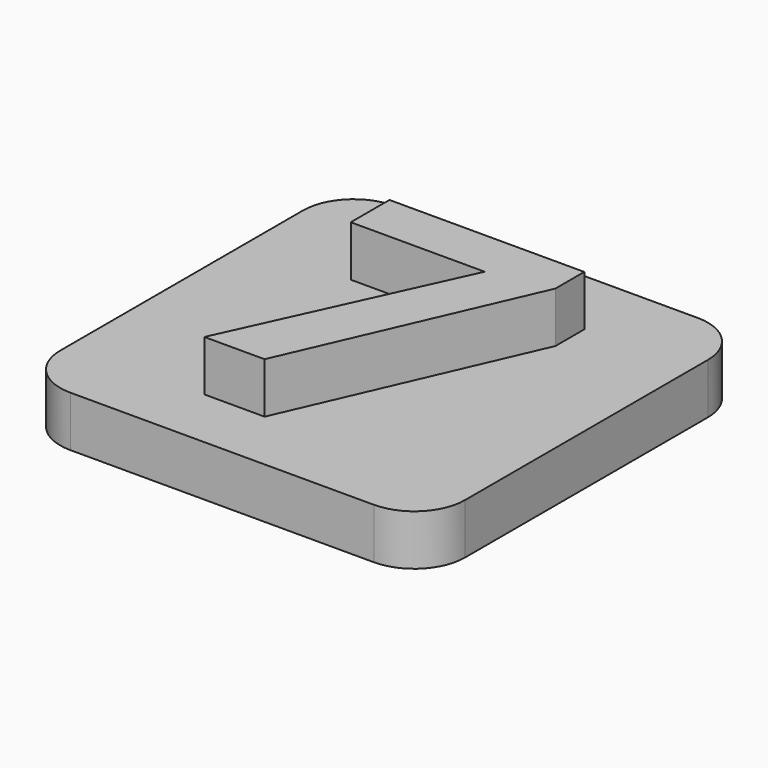
from build123d import *

# Parameters (mm, degrees)
F1_DEPTH     = 6.35
F2_TEXT_SIZE = 47.7457212077
F3_DEPTH     = 6.35


# Not quite as in the source:
# - Text() gives the source's letters only with a copy of the font that has no kerning and outlines rounded to 1/6400 em; it was checked with that copy


with BuildPart() as f1:
    # F0 (on Top) → F1 (new body)
    with BuildSketch(Plane.XY):
        with BuildLine():
            Line((-10.4569760919, 61.7519390389), (-48.5569760919, 61.7519390389))
            ThreePointArc((-48.5569760919, 61.7519390389), (-53.0471041524, 59.8920670995), (-54.9069760919, 55.4019390389))
            Line((-54.9069760919, 55.4019390389), (-54.9069760919, 17.3019390389))
            ThreePointArc((-54.9069760919, 17.3019390389), (-53.0471041524, 12.8118109784), (-48.5569760919, 10.9519390389))
            Line((-48.5569760919, 10.9519390389), (-10.4569760919, 10.9519390389))
            ThreePointArc((-10.4569760919, 10.9519390389), (-5.9668480313, 12.8118109784), (-4.1069760919, 17.3019390389))
            Line((-4.1069760919, 17.3019390389), (-4.1069760919, 55.4019390389))
            ThreePointArc((-4.1069760919, 55.4019390389), (-5.9668480313, 59.8920670995), (-10.4569760919, 61.7519390389))
        make_face()
    extrude(amount=F1_DEPTH)

    # F2 (on face) → F3 (join)
    with BuildSketch(Plane.XY.offset(6.35)):
        with Locations((-43.3514267206, 18.8616737723)):
            Text('7', F2_TEXT_SIZE, font='Open Sans', font_style=FontStyle.BOLD, text_align=(TextAlign.LEFT, TextAlign.BOTTOM))
    extrude(amount=F3_DEPTH)


solid = f1.part
